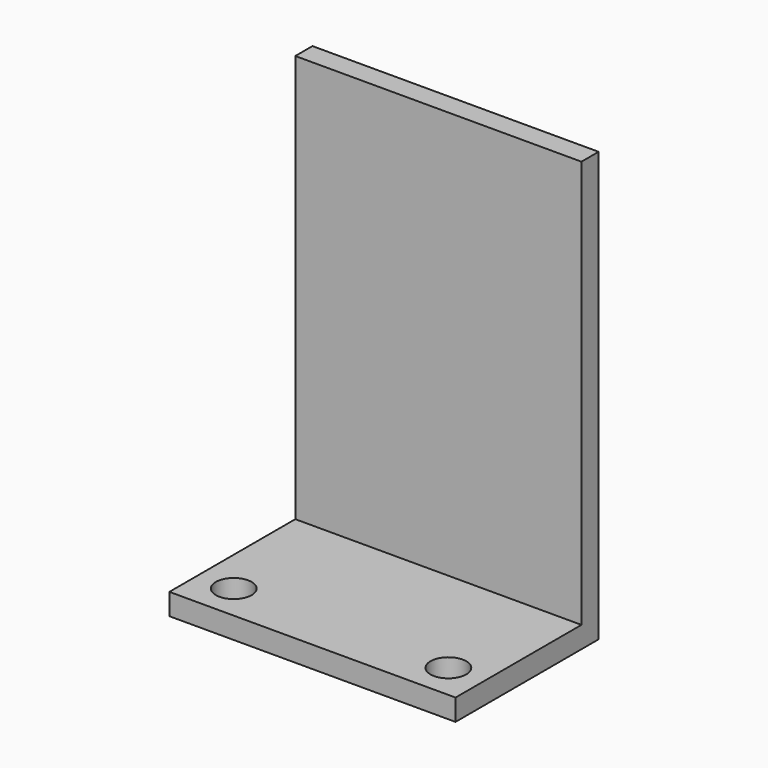
from build123d import *

# Parameters (mm, degrees)
F1_DEPTH = 80
F3_D     = 10


# Not quite as in the source:
# - a feature names something its author has since deleted; it is built from what else it names


with BuildPart() as f1:
    # F0 (on Right) → F1 (new body)
    with BuildSketch(Plane.YZ):
        Polygon((0, 0), (0, 120), (-6, 120), (-6, 6), (-50, 6), (-50, 0), align=None)
    extrude(amount=F1_DEPTH)

    # F3 (through all)
    with Locations(Plane(origin=(0, 0, 0), x_dir=(1, 0, 0), z_dir=(0, 0, -1))):
        with Locations((10, 40), (70, 40)):
            Hole(F3_D / 2)


solid = f1.part
